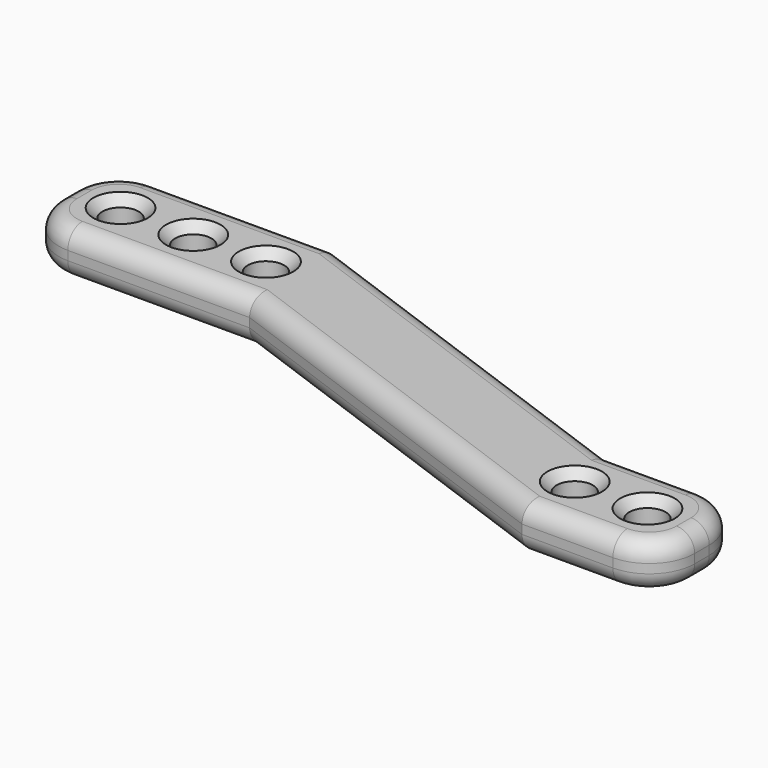
from build123d import *

# Parameters (mm, degrees)
F0_W         = 25
F0_H         = 12
F0_W_2       = 15
F1_DEPTH     = 5
F2_R         = 2
F3_DEPTH     = 5.001
F4_R         = 2
F5_T1_DEPTH  = 5
F5_T4_ANGLE  = 90
F5_T6_ANGLE  = 90
F5_T8_ANGLE  = 90
F5_T10_ANGLE = 90
F5_T12_ANGLE = 90
F5_T14_ANGLE = 90
F5_T16_ANGLE = 90
F5_T18_ANGLE = 90
F6_SIZE      = 1


# Not quite as in the source:
# - a fillet or chamfer that OpenCascade refuses, or shapes differently, is made with other operations: its cross-section is extruded or revolved along the edge and cut away or added


with BuildPart() as f1:
    # F0 (on Top) → F1 (new body)
    with BuildSketch(Plane.XY):
        with Locations((12.5, -6)):
            Rectangle(F0_W, F0_H)
        Polygon((67.2861679354, -15.3909064497), (25, 0), (25, -12), (67.2861679354, -27.3909064497), align=None)
        with Locations((74.7861679354, -21.3909064497)):
            Rectangle(F0_W_2, F0_H)
    extrude(amount=F1_DEPTH)

    # F2 (on face) → F3 (cut, through all)
    with BuildSketch(Plane.XY.offset(5)):
        with Locations((6, -6)):
            Circle(F2_R)
        with Locations((76.2861679354, -21.3909064497)):
            Circle(F2_R)
        with Locations((14, -6)):
            Circle(F2_R)
        with Locations((22, -6)):
            Circle(F2_R)
        with Locations((68.2861679354, -21.3909064497)):
            Circle(F2_R)
    extrude(amount=-F3_DEPTH, mode=Mode.SUBTRACT)

    # F4
    f4_edges = [f1.edges().sort_by_distance(p)[0] for p in [
        (46.143084, -7.695453, 5),
        (74.786168, -15.390906, 5),
        (82.286168, -21.390906, 5),
        (74.786168, -27.390906, 5),
        (46.143084, -19.695453, 5),
        (12.5, -12, 5),
        (0, -6, 5),
        (12.5, 0, 5),
        (12.5, -12, 0),
        (0, -6, 0),
        (12.5, 0, 0),
        (46.143084, -7.695453, 0),
        (46.143084, -19.695453, 0),
        (74.786168, -27.390906, 0),
        (74.786168, -15.390906, 0),
        (82.286168, -21.390906, 0),
    ]]
    fillet(f4_edges, radius=F4_R)

    # F5: fillet of radius 5 on 4 edges, made by hand

    # F5_s2 → F5_t1 (cut)
    with BuildSketch(Plane.XY):
        with BuildLine():
            ThreePointArc((77.2861679354, -15.3909064497), (80.8217018413, -16.8553725437), (82.2861679354, -20.3909064497))
            Line((82.2861679354, -20.3909064497), (82.2861679354, -15.3909064497))
            Line((82.2861679354, -15.3909064497), (77.2861679354, -15.3909064497))
        make_face()
        with BuildLine():
            ThreePointArc((82.2861679354, -22.3909064497), (80.8217018413, -25.9264403556), (77.2861679354, -27.3909064497))
            Line((77.2861679354, -27.3909064497), (82.2861679354, -27.3909064497))
            Line((82.2861679354, -27.3909064497), (82.2861679354, -22.3909064497))
        make_face()
        with BuildLine():
            ThreePointArc((0, -7), (1.4644660941, -10.5355339059), (5, -12))
            Line((5, -12), (0, -12))
            Line((0, -12), (0, -7))
        make_face()
        with BuildLine():
            ThreePointArc((5, 0), (1.4644660941, -1.4644660941), (0, -5))
            Line((0, -5), (0, 0))
            Line((0, 0), (5, 0))
        make_face()
    extrude(amount=F5_T1_DEPTH, mode=Mode.SUBTRACT)

    # F5_s3 → F5_t4 (revolve, cut)
    with BuildSketch(Plane.XZ.offset(5)):
        with BuildLine():
            ThreePointArc((2, 0), (0.5857864376, 0.5857864376), (0, 2))
            Line((0, 2), (0, 0))
            Line((0, 0), (2, 0))
        make_face()
    revolve(axis=Axis((5, -5, 0), (0, 0, -1)), revolution_arc=F5_T4_ANGLE, mode=Mode.SUBTRACT)

    # F5_s5 → F5_t6 (revolve, cut)
    with BuildSketch(Plane.YZ.offset(5)):
        with BuildLine():
            ThreePointArc((-10, 0), (-11.4142135624, 0.5857864376), (-12, 2))
            Line((-12, 2), (-12, 0))
            Line((-12, 0), (-10, 0))
        make_face()
    revolve(axis=Axis((5, -7, 0), (0, 0, -1)), revolution_arc=F5_T6_ANGLE, mode=Mode.SUBTRACT)

    # F5_s7 → F5_t8 (revolve, cut)
    with BuildSketch(Plane.XZ.offset(22.3909064497)):
        with BuildLine():
            ThreePointArc((80.2861679354, 0), (81.7003814977, 0.5857864376), (82.2861679354, 2))
            Line((82.2861679354, 2), (82.2861679354, 0))
            Line((82.2861679354, 0), (80.2861679354, 0))
        make_face()
    revolve(axis=Axis((77.2861679354, -22.3909064497, 0), (0, 0, -1)), revolution_arc=F5_T8_ANGLE, mode=Mode.SUBTRACT)

    # F5_s9 → F5_t10 (revolve, cut)
    with BuildSketch(Plane.YZ.offset(77.2861679354)):
        with BuildLine():
            ThreePointArc((-17.3909064497, 0), (-15.9766928873, 0.5857864376), (-15.3909064497, 2))
            Line((-15.3909064497, 2), (-15.3909064497, 0))
            Line((-15.3909064497, 0), (-17.3909064497, 0))
        make_face()
    revolve(axis=Axis((77.2861679354, -20.3909064497, 0), (0, 0, -1)), revolution_arc=F5_T10_ANGLE, mode=Mode.SUBTRACT)

    # F5_s11 → F5_t12 (revolve, cut)
    with BuildSketch(Plane.XZ.offset(20.3909064497)):
        with BuildLine():
            ThreePointArc((80.2861679354, 5), (81.7003814977, 4.4142135624), (82.2861679354, 3))
            Line((82.2861679354, 3), (82.2861679354, 5))
            Line((82.2861679354, 5), (80.2861679354, 5))
        make_face()
    revolve(axis=Axis((77.2861679354, -20.3909064497, 5), (0, 0, 1)), revolution_arc=F5_T12_ANGLE, mode=Mode.SUBTRACT)

    # F5_s13 → F5_t14 (revolve, cut)
    with BuildSketch(Plane.YZ.offset(77.2861679354)):
        with BuildLine():
            ThreePointArc((-25.3909064497, 5), (-26.805120012, 4.4142135624), (-27.3909064497, 3))
            Line((-27.3909064497, 3), (-27.3909064497, 5))
            Line((-27.3909064497, 5), (-25.3909064497, 5))
        make_face()
    revolve(axis=Axis((77.2861679354, -22.3909064497, 5), (0, 0, 1)), revolution_arc=F5_T14_ANGLE, mode=Mode.SUBTRACT)

    # F5_s15 → F5_t16 (revolve, cut)
    with BuildSketch(Plane.XZ.offset(7)):
        with BuildLine():
            ThreePointArc((2, 5), (0.5857864376, 4.4142135624), (0, 3))
            Line((0, 3), (0, 5))
            Line((0, 5), (2, 5))
        make_face()
    revolve(axis=Axis((5, -7, 5), (0, 0, 1)), revolution_arc=F5_T16_ANGLE, mode=Mode.SUBTRACT)

    # F5_s17 → F5_t18 (revolve, cut)
    with BuildSketch(Plane.YZ.offset(5)):
        with BuildLine():
            ThreePointArc((-2, 5), (-0.5857864376, 4.4142135624), (0, 3))
            Line((0, 3), (0, 5))
            Line((0, 5), (-2, 5))
        make_face()
    revolve(axis=Axis((5, -5, 5), (0, 0, 1)), revolution_arc=F5_T18_ANGLE, mode=Mode.SUBTRACT)

    # F6
    f6_edges = [f1.edges().sort_by_distance(p)[0] for p in [
        (20, -6, 5),
        (24, -6, 2.5),
        (20, -6, 0),
        (12, -6, 5),
        (16, -6, 2.5),
        (12, -6, 0),
        (4, -6, 5),
        (8, -6, 2.5),
        (4, -6, 0),
        (66.286168, -21.390906, 5),
        (70.286168, -21.390906, 2.5),
        (66.286168, -21.390906, 0),
        (74.286168, -21.390906, 5),
        (78.286168, -21.390906, 2.5),
        (74.286168, -21.390906, 0),
    ]]
    chamfer(f6_edges, length=F6_SIZE)


solid = f1.part
